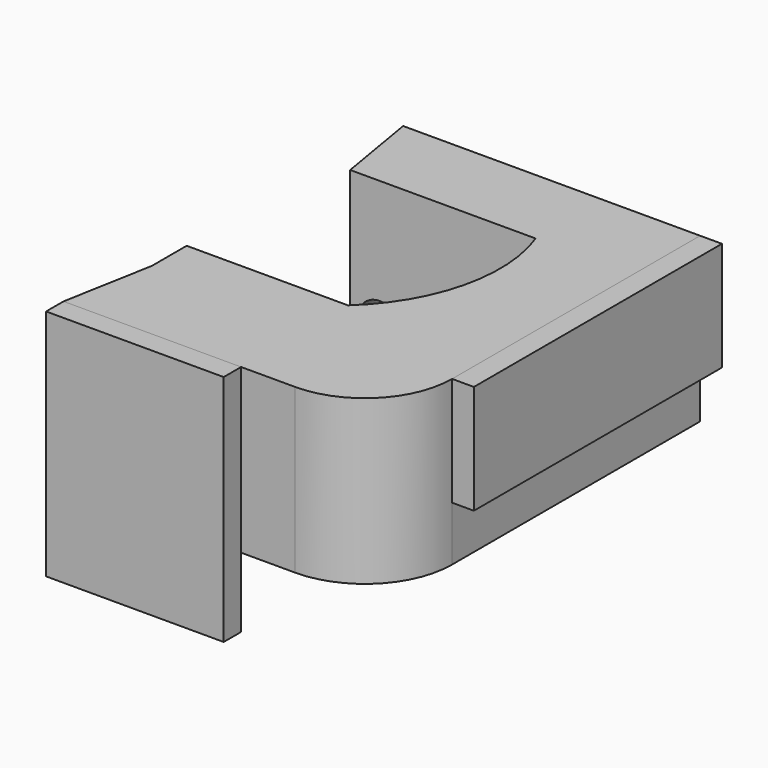
from build123d import *

# Parameters (mm, degrees)
F0_W      = 2
F0_H      = 28.4474462867
F1_DEPTH  = 10
F2_DEPTH  = 21.4
F3_DEPTH  = 15
F4_R      = 2
F5_DEPTH  = 8
F4_R_2    = 2.1
F6_DEPTH  = 5
F4_R_3    = 2.2
F7_DEPTH  = 4.5
F4_R_4    = 2.3
F8_DEPTH  = 4
F4_R_5    = 2.4
F9_DEPTH  = 3.5
F4_R_6    = 2.5
F10_DEPTH = 3
F4_R_7    = 2.6
F11_DEPTH = 2.5
F4_R_8    = 2.7
F12_DEPTH = 2
F4_R_9    = 2.8
F13_DEPTH = 1.5
F4_R_10   = 2.9
F14_DEPTH = 1
F4_R_11   = 3
F15_DEPTH = 0.5
F16_R     = 2
F17_DEPTH = 15


with BuildPart() as f1:
    # F0 (on Top) → F1 (new body)
    with BuildSketch(Plane.XY):
        with Locations((24.25, -1.2762768567)):
            Rectangle(F0_W, F0_H)
    extrude(amount=-F1_DEPTH)


with BuildPart() as f2:
    # F0 (on Top) → F2 (new body)
    with BuildSketch(Plane.XY):
        Polygon((0, -23.5), (-6, -23.5), (-6, -25.5), (10.295630141, -25.5), (10.295630141, -23.5), align=None)
    extrude(amount=-F2_DEPTH)


with BuildPart() as f3:
    # F0 (on Top) → F3 (new body)
    with BuildSketch(Plane.XY):
        with BuildLine():
            ThreePointArc((10.295630141, -11.25), (5.5226805086, -14.2148689758), (0, -15.25))
            Line((0, -15.25), (-4.5, -15.25))
            Line((-4.5, -15.25), (-6, -23.5))
            Line((-6, -23.5), (0, -23.5))
            Line((0, -23.5), (10.295630141, -23.5))
            Line((10.295630141, -23.5), (15.25, -23.5))
            ThreePointArc((15.25, -23.5), (20.9068542495, -21.1568542495), (23.25, -15.5))
            Line((23.25, -15.5), (23.25, 12.9474462867))
            Line((23.25, 12.9474462867), (8.0576755118, 12.9474462867))
            ThreePointArc((8.0576755118, 12.9474462867), (11.8312459859, 9.6220641455), (14.3178210633, 5.25))
            ThreePointArc((14.3178210633, 5.25), (14.816139681, -3.611717729), (10.295630141, -11.25))
        make_face()
        with BuildLine():
            Line((-4.5, -15.25), (0, -15.25))
            ThreePointArc((0, -15.25), (5.5226805086, -14.2148689758), (10.295630141, -11.25))
            Line((10.295630141, -11.25), (0, -11.25))
            Line((0, -11.25), (-4.5, -13.75))
            Line((-4.5, -13.75), (-4.5, -15.25))
        make_face()
        with BuildLine():
            Line((2.7, 5.25), (14.3178210633, 5.25))
            ThreePointArc((14.3178210633, 5.25), (11.8312459859, 9.6220641455), (8.0576755118, 12.9474462867))
            Line((8.0576755118, 12.9474462867), (4, 12.9474462867))
            Line((4, 12.9474462867), (2.7, 5.25))
        make_face()
        Polygon((-2.7, 5.25), (2.7, 5.25), (4, 12.9474462867), (-4, 12.9474462867), align=None)
        Polygon((-4.5, -13.75), (0, -11.25), (-4.5, -11.25), align=None)
    extrude(amount=-F3_DEPTH)

    # F4 (on face) → F5 (cut)
    with BuildSketch(Plane(origin=(0, 12.9474462867, 0), x_dir=(-1, 0, 0), z_dir=(0, 1, 0))):
        with Locations((0, -11.7)):
            Circle(F4_R)
    extrude(amount=-F5_DEPTH, mode=Mode.SUBTRACT)

    # F4 (on face) → F6 (cut)
    with BuildSketch(Plane(origin=(0, 12.9474462867, 0), x_dir=(-1, 0, 0), z_dir=(0, 1, 0))):
        with Locations((0, -11.7)):
            Circle(F4_R_2)
        with Locations((0, -11.7)):
            Circle(F4_R, mode=Mode.SUBTRACT)
    extrude(amount=-F6_DEPTH, mode=Mode.SUBTRACT)

    # F4 (on face) → F7 (cut)
    with BuildSketch(Plane(origin=(0, 12.9474462867, 0), x_dir=(-1, 0, 0), z_dir=(0, 1, 0))):
        with Locations((0, -11.7)):
            Circle(F4_R_3)
        with Locations((0, -11.7)):
            Circle(F4_R_2, mode=Mode.SUBTRACT)
    extrude(amount=-F7_DEPTH, mode=Mode.SUBTRACT)

    # F4 (on face) → F8 (cut)
    with BuildSketch(Plane(origin=(0, 12.9474462867, 0), x_dir=(-1, 0, 0), z_dir=(0, 1, 0))):
        with Locations((0, -11.7)):
            Circle(F4_R_4)
        with Locations((0, -11.7)):
            Circle(F4_R_3, mode=Mode.SUBTRACT)
    extrude(amount=-F8_DEPTH, mode=Mode.SUBTRACT)

    # F4 (on face) → F9 (cut)
    with BuildSketch(Plane(origin=(0, 12.9474462867, 0), x_dir=(-1, 0, 0), z_dir=(0, 1, 0))):
        with Locations((0, -11.7)):
            Circle(F4_R_5)
        with Locations((0, -11.7)):
            Circle(F4_R_4, mode=Mode.SUBTRACT)
    extrude(amount=-F9_DEPTH, mode=Mode.SUBTRACT)

    # F4 (on face) → F10 (cut)
    with BuildSketch(Plane(origin=(0, 12.9474462867, 0), x_dir=(-1, 0, 0), z_dir=(0, 1, 0))):
        with Locations((0, -11.7)):
            Circle(F4_R_6)
        with Locations((0, -11.7)):
            Circle(F4_R_5, mode=Mode.SUBTRACT)
    extrude(amount=-F10_DEPTH, mode=Mode.SUBTRACT)

    # F4 (on face) → F11 (cut)
    with BuildSketch(Plane(origin=(0, 12.9474462867, 0), x_dir=(-1, 0, 0), z_dir=(0, 1, 0))):
        with Locations((0, -11.7)):
            Circle(F4_R_7)
        with Locations((0, -11.7)):
            Circle(F4_R_6, mode=Mode.SUBTRACT)
    extrude(amount=-F11_DEPTH, mode=Mode.SUBTRACT)

    # F4 (on face) → F12 (cut)
    with BuildSketch(Plane(origin=(0, 12.9474462867, 0), x_dir=(-1, 0, 0), z_dir=(0, 1, 0))):
        with Locations((0, -11.7)):
            Circle(F4_R_8)
        with Locations((0, -11.7)):
            Circle(F4_R_7, mode=Mode.SUBTRACT)
    extrude(amount=-F12_DEPTH, mode=Mode.SUBTRACT)

    # F4 (on face) → F13 (cut)
    with BuildSketch(Plane(origin=(0, 12.9474462867, 0), x_dir=(-1, 0, 0), z_dir=(0, 1, 0))):
        with Locations((0, -11.7)):
            Circle(F4_R_9)
        with Locations((0, -11.7)):
            Circle(F4_R_8, mode=Mode.SUBTRACT)
    extrude(amount=-F13_DEPTH, mode=Mode.SUBTRACT)

    # F4 (on face) → F14 (cut)
    with BuildSketch(Plane(origin=(0, 12.9474462867, 0), x_dir=(-1, 0, 0), z_dir=(0, 1, 0))):
        with Locations((0, -11.7)):
            Circle(F4_R_10)
        with Locations((0, -11.7)):
            Circle(F4_R_9, mode=Mode.SUBTRACT)
    extrude(amount=-F14_DEPTH, mode=Mode.SUBTRACT)

    # F4 (on face) → F15 (cut)
    with BuildSketch(Plane(origin=(0, 12.9474462867, 0), x_dir=(-1, 0, 0), z_dir=(0, 1, 0))):
        with Locations((0, -11.7)):
            Circle(F4_R_11)
        with Locations((0, -11.7)):
            Circle(F4_R_10, mode=Mode.SUBTRACT)
    extrude(amount=-F15_DEPTH, mode=Mode.SUBTRACT)

    # F16 (on face) → F17 (cut)
    with BuildSketch(Plane(origin=(0, -11.25, 0), x_dir=(-1, 0, 0), z_dir=(0, 1, 0))):
        with Locations((0, -11.7)):
            Circle(F16_R)
    extrude(amount=-F17_DEPTH, mode=Mode.SUBTRACT)


solid = Compound([f1.part, f2.part, f3.part])
